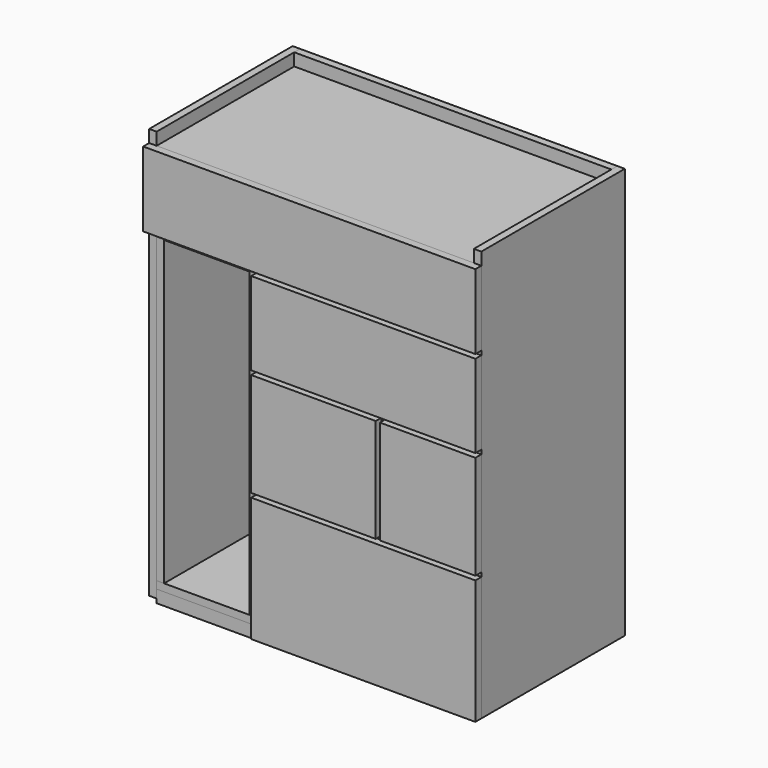
from build123d import *

# Parameters (mm, degrees)
F0_W          = 18
F0_H          = 414
F0_H_2        = 18
F1_DEPTH      = 990
F0_W_2        = 764
F2_DEPTH      = 990
F3_DEPTH      = 20
F3_DEPTH_BACK = 10
F4_W          = 782
F4_H          = 180
F4_W_2        = 18
F5_DEPTH      = 18
F4_W_3        = 540
F4_H_2        = 200
F4_W_4        = 230
F4_H_3        = 250
F4_H_4        = 300
F4_W_5        = 300
F6_W          = 764
F6_H          = 18
F7_DEPTH      = 414
F6_H_2        = 4
F6_W_2        = 18
F6_W_3        = 206
F6_H_3        = 192
F6_H_4        = 258
F6_H_5        = 242
F8_DEPTH      = 414
F9_R          = 10
F10_DEPTH     = 206
F11_W         = 206
F11_H         = 728
F12_DEPTH     = 12


# Not quite as in the source:
# - a feature names something its author has since deleted; it is built from what else it names


with BuildPart() as f1:
    # F0 (on Top) → F1 (new body)
    with BuildSketch(Plane.XY):
        with Locations((9, 207)):
            Rectangle(F0_W, F0_H)
        with Locations((9, 423)):
            Rectangle(F0_W, F0_H_2)
    extrude(amount=F1_DEPTH)


with BuildPart() as f1b:
    # F0 (on Top) → F1, piece 2 (new body)
    with BuildSketch(Plane.XY):
        with Locations((791, 423)):
            Rectangle(F0_W, F0_H_2)
        with Locations((791, 207)):
            Rectangle(F0_W, F0_H)
    extrude(amount=F1_DEPTH)


with BuildPart() as f2:
    # F0 (on Top) → F2 (new body, through all)
    with BuildSketch(Plane.XY):
        with Locations((400, 423)):
            Rectangle(F0_W_2, F0_H_2)
    extrude(amount=F2_DEPTH)


with BuildPart() as f3:
    # F0 (on Top) → F3 (new body, two sides)
    with BuildSketch(Plane.XY) as f3_sk:
        with Locations((400, 207)):
            Rectangle(F0_W_2, F0_H)
    extrude(amount=F3_DEPTH)
    extrude(f3_sk.sketch, amount=-F3_DEPTH_BACK)


with BuildPart() as f5:
    # F4 (on face) → F5 (new body)
    with BuildSketch(Plane.XZ):
        with Locations((409, 870)):
            Rectangle(F4_W, F4_H)
        with Locations((9, 870)):
            Rectangle(F4_W_2, F4_H)
    extrude(amount=F5_DEPTH)


with BuildPart() as f5b:
    # F4 (on face) → F5, piece 2 (new body)
    with BuildSketch(Plane.XZ):
        with Locations((530, 670)):
            Rectangle(F4_W_3, F4_H_2)
    extrude(amount=F5_DEPTH)


with BuildPart() as f5c:
    # F4 (on face) → F5, piece 3 (new body)
    with BuildSketch(Plane.XZ):
        with Locations((685, 435)):
            Rectangle(F4_W_4, F4_H_3)
    extrude(amount=F5_DEPTH)


with BuildPart() as f5d:
    # F4 (on face) → F5, piece 4 (new body)
    with BuildSketch(Plane.XZ):
        with Locations((530, 150)):
            Rectangle(F4_W_3, F4_H_4)
    extrude(amount=F5_DEPTH)


with BuildPart() as f5e:
    # F4 (on face) → F5, piece 5 (new body)
    with BuildSketch(Plane.XZ):
        with Locations((410, 435)):
            Rectangle(F4_W_5, F4_H_3)
    extrude(amount=F5_DEPTH)


with BuildPart() as f7:
    # F6 (on face) → F7 (new body, through all)
    with BuildSketch(Plane(origin=(0, 0, 0), x_dir=(-1, 0, 0), z_dir=(0, 1, 0))):
        with Locations((-400, 951)):
            Rectangle(F6_W, F6_H)
    extrude(amount=F7_DEPTH)


with BuildPart() as f7b:
    # F6 (on face) → F7, piece 2 (new body, through all)
    with BuildSketch(Plane(origin=(0, 0, 0), x_dir=(-1, 0, 0), z_dir=(0, 1, 0))):
        Polygon((-18, 780), (-782, 780), (-782, 766), (-260, 766), (-242, 766), (-36, 766), (-18, 766), align=None)
        with Locations((-400, 782)):
            Rectangle(F6_W, F6_H_2)
    extrude(amount=F7_DEPTH)


with BuildPart() as f7c:
    # F6 (on face) → F7, piece 3 (new body, through all)
    with BuildSketch(Plane(origin=(0, 0, 0), x_dir=(-1, 0, 0), z_dir=(0, 1, 0))):
        Polygon((-260, 556), (-260, 574), (-782, 574), (-782, 556), (-574, 556), (-556, 556), align=None)
    extrude(amount=F7_DEPTH)


with BuildPart() as f7d:
    # F6 (on face) → F7, piece 4 (new body, through all)
    with BuildSketch(Plane(origin=(0, 0, 0), x_dir=(-1, 0, 0), z_dir=(0, 1, 0))):
        Polygon((-260, 296), (-260, 314), (-556, 314), (-574, 314), (-782, 314), (-782, 296), align=None)
    extrude(amount=F7_DEPTH)


with BuildPart() as f7e:
    # F6 (on face) → F7, piece 5 (new body, through all)
    with BuildSketch(Plane(origin=(0, 0, 0), x_dir=(-1, 0, 0), z_dir=(0, 1, 0))):
        with Locations((-251, 29)):
            Rectangle(F6_W_2, F6_H)
        with Locations((-139, 29)):
            Rectangle(F6_W_3, F6_H)
        with Locations((-27, 29)):
            Rectangle(F6_W_2, F6_H)
    extrude(amount=F7_DEPTH)


with BuildPart() as f8:
    # F6 (on face) → F8 (new body, through all)
    with BuildSketch(Plane(origin=(0, 0, 0), x_dir=(-1, 0, 0), z_dir=(0, 1, 0))):
        with Locations((-251, 670)):
            Rectangle(F6_W_2, F6_H_3)
        with Locations((-251, 167)):
            Rectangle(F6_W_2, F6_H_4)
        with Locations((-251, 305)):
            Rectangle(F6_W_2, F6_H)
        with Locations((-251, 435)):
            Rectangle(F6_W_2, F6_H_5)
        with Locations((-251, 565)):
            Rectangle(F6_W_2, F6_H)
    extrude(amount=F8_DEPTH)


with BuildPart() as f8b:
    # F6 (on face) → F8, piece 2 (new body, through all)
    with BuildSketch(Plane(origin=(0, 0, 0), x_dir=(-1, 0, 0), z_dir=(0, 1, 0))):
        with Locations((-565, 435)):
            Rectangle(F6_W_2, F6_H_5)
    extrude(amount=F8_DEPTH)


with BuildPart() as f8c:
    # F6 (on face) → F8, piece 3 (new body, through all)
    with BuildSketch(Plane(origin=(0, 0, 0), x_dir=(-1, 0, 0), z_dir=(0, 1, 0))):
        with Locations((-27, 670)):
            Rectangle(F6_W_2, F6_H_3)
        with Locations((-27, 565)):
            Rectangle(F6_W_2, F6_H)
        with Locations((-27, 435)):
            Rectangle(F6_W_2, F6_H_5)
        with Locations((-27, 305)):
            Rectangle(F6_W_2, F6_H)
        with Locations((-27, 167)):
            Rectangle(F6_W_2, F6_H_4)
    extrude(amount=F8_DEPTH)


with BuildPart() as f10:
    # F9 (on face) → F10 (new body, through all)
    with BuildSketch(Plane.YZ.offset(36)):
        with Locations((207, 706)):
            Circle(F9_R)
    extrude(amount=F10_DEPTH)


with BuildPart() as f12:
    # F11 (on face) → F12 (new body)
    with BuildSketch(Plane.XZ.offset(-414)):
        with Locations((139, 402)):
            Rectangle(F11_W, F11_H)
    extrude(amount=F12_DEPTH)


solid = Compound([f1.part, f1b.part, f2.part, f3.part, f5.part, f5b.part, f5c.part, f5d.part, f5e.part, f7.part, f7b.part, f7c.part, f7d.part, f7e.part, f8.part, f8b.part, f8c.part, f10.part, f12.part])
